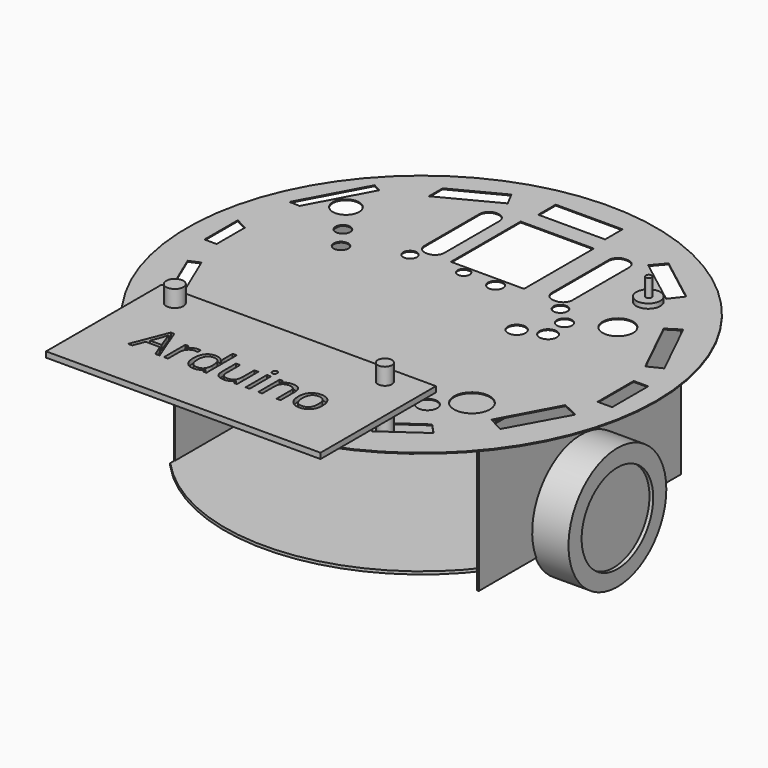
from build123d import *

# Parameters (mm, degrees)
F0_R           = 63.9111702995
F1_DEPTH       = 0.254
F2_W           = 18.2276954874
F2_H           = 5.9562139213
F2_W_2         = 3.9726644754
F2_H_2         = 12.3111242428
F2_W_3         = 18.6114357784
F2_H_3         = 3.4572258592
F2_W_4         = 19.9545305222
F2_H_4         = 23.7919427454
F2_R           = 1.6505332981
F2_R_2         = 2.0396113473
F2_W_5         = 5.3723761812
F2_H_5         = 23.7919408828
F2_W_6         = 5.5642463267
F2_H_6         = 24.3675541133
F2_R_3         = 1.8501413146
F2_R_4         = 1.8832977576
F2_R_5         = 2.0535644144
F2_R_6         = 2.3408672102
F2_R_7         = 2.3992175774
F2_R_8         = 2.0043342178
F2_R_9         = 3.5959734762
F2_R_10        = 1.9777561013
F2_R_11        = 4.047513939
F2_R_12        = 1.9567032502
F2_R_13        = 1.9754290284
F2_R_14        = 4.8842283694
F2_R_15        = 2.6724465659
F2_R_16        = 2.5813546875
F2_R_17        = 4.1507926028
F3_DEPTH       = 53.34
F3_DEPTH_BACK  = 76.454
F4_R           = 3.2674386057
F5_DEPTH       = 1.524
F6_R           = 0.777196863
F7_DEPTH       = 6.35
F8_R           = 2.54
F9_R           = 2.3420782562
F9_R_2         = 1.9282730437
F10_DEPTH      = 15.748
F10_DEPTH_BACK = 2.794
F12_START      = 9.652
F11_W          = 74.8294964433
F11_H          = 39.3334552646
F12_DEPTH      = 1.524
F14_START      = 9.906
F13_TEXT_SIZE  = 13.6177572939
F14_DEPTH      = 10.668
F16_START      = 42.926
F15_W          = 68.8815116882
F15_H          = 37.894424051
F16_DEPTH      = 0.508
F18_START      = -39.37
F17_W          = 69.0733827651
F17_H          = 38.0862951279
F18_DEPTH      = 0.254
F20_START      = 43.18
F19_R          = 16.6703050867
F20_DEPTH      = 10.16
F22_START      = -39.4462
F21_R          = 16.5595980484
F22_DEPTH      = 7.5438
F24_START      = 52.324
F23_R          = 12.195203819
F24_DEPTH      = 51.816
F26_START      = -44.958
F25_R          = 11.3790282157
F26_DEPTH      = 13.208
F28_START      = -33.528
F27_R          = 53.684976613
F28_DEPTH      = 0.762
F30_START      = -29.718
F30_DEPTH      = 27.432
F31_W          = 27.6789963245
F31_H          = 85.5889506638
F32_DEPTH      = 57.658
F32_DEPTH_BACK = 47.244


# Not quite as in the source:
# - Text() gives the source's letters only with a copy of the font that has no kerning and outlines rounded to 1/6400 em; it was checked with that copy


with BuildPart() as f1:
    # F0 (on Top) → F1 (new body)
    with BuildSketch(Plane.XY):
        Circle(F0_R)
    extrude(amount=F1_DEPTH)

    # F2 (on Top) → F3 (cut, two sides)
    with BuildSketch(Plane.XY) as f3_sk:
        with Locations((-0.1918715425, 54.2952399701)):
            Rectangle(F2_W, F2_H)
        Polygon((38.8790406287, 41.5468643842), (26.382194832, 51.1334910989), (23.5169891404, 47.7691923058), (36.192856729, 38.0452337299), align=None)
        Polygon((55.930249393, 12.7593884245), (47.8716939688, 29.2602516711), (44.3243973017, 27.0042982848), (52.1765033906, 10.9261649284), align=None)
        with Locations((56.4382374287, -1.9989344291)):
            Rectangle(F2_W_2, F2_H_2)
        Polygon((46.0938289762, -30.9211090207), (54.4519051909, -15.7124722151), (50.0560939326, -13.6060078889), (41.9458702218, -28.691023613), align=None)
        Polygon((25.3998646187, -48.7983639411), (36.192856729, -41.2095412612), (33.4562764833, -38.2781662047), (23.1152811685, -45.5491786335), align=None)
        with Locations((-0.383741688, -53.8179017603)):
            Rectangle(F2_W_3, F2_H_3)
        Polygon((-42.1155765653, -38.2781662047), (-30.0277341157, -49.5985262096), (-27.4126883596, -45.6261113286), (-38.795024669, -34.7324920255), align=None)
        Polygon((-54.3377436697, -11.8860941993), (-48.9752166669, -24.5263342954), (-46.2652777131, -23.0668127871), (-51.5164032923, -10.6891617167), align=None)
        Polygon((-57.6570853591, 9.3794129285), (-57.6570853591, -2.014640253), (-54.3377436697, -2.014640253), (-54.3377436697, 7.5948205777), align=None)
        Polygon((-44.993635267, 40.1968695223), (-54.3377436697, 22.8168283287), (-51.5164032923, 22.7366536856), (-42.7715001208, 39.0021731772), align=None)
        Polygon((-19.5502191782, 54.9985840917), (-32.8018183124, 48.1027527126), (-32.8018183124, 43.4243921615), (-17.6344756037, 51.3171330094), align=None)
        with Locations((-0.2878075466, 34.6326250583)):
            Rectangle(F2_W_4, F2_H_4)
        with Locations((-5.0845686346, 20.6260792911)):
            Circle(F2_R)
        with Locations((3.933345899, 20.2423390001)):
            Circle(F2_R_2)
        with Locations((-16.5967992507, 34.4407549128)):
            Rectangle(F2_W_5, F2_H_5)
        with Locations((18.2276982814, 34.728561528)):
            Rectangle(F2_W_6, F2_H_6)
        with Locations((-19.0911162645, 19.8585987091)):
            Circle(F2_R_3)
        with Locations((21.5149857104, 20.3715078533)):
            Circle(F2_R_4)
        with Locations((26.1894725263, 15.9154105932)):
            Circle(F2_R_5)
        with Locations((26.7599057406, 9.5835877582)):
            Circle(F2_R_6)
        with Locations((20.2569533139, 7.0166331716)):
            Circle(F2_R_7)
        with Locations((-37.5732146204, 20.0800783932)):
            Circle(F2_R_8)
        with Locations((-43.4749871492, 28.491800651)):
            Circle(F2_R_9)
        with Locations((-33.0960080028, 13.8391247019)):
            Circle(F2_R_10)
        with Locations((-24.6553607285, -30.7952146977)):
            Circle(F2_R_11)
        with Locations((-17.9398916662, -38.0862951279)):
            Circle(F2_R_12)
        with Locations((-5.8520506136, -30.2196051925)):
            Circle(F2_R_13)
        with Locations((33.8651463389, -25.2309720963)):
            Circle(F2_R_14)
        with Locations((26.9578043371, -31.7545682192)):
            Circle(F2_R_15)
        with Locations((20.2423371375, -29.2602516711)):
            Circle(F2_R_16)
        with Locations((36.3594591618, 21.3935598731)):
            Circle(F2_R_17)
    extrude(amount=F3_DEPTH, mode=Mode.SUBTRACT)
    extrude(f3_sk.sketch, amount=-F3_DEPTH_BACK, mode=Mode.SUBTRACT)

    # F4 (on Top) → F5 (join)
    with BuildSketch(Plane.XY):
        with Locations((34.0570136905, 34.6326269209)):
            Circle(F4_R)
    extrude(amount=F5_DEPTH)

    # F6 (on Top) → F7 (join)
    with BuildSketch(Plane.XY):
        with Locations((34.1490767896, 34.6543379128)):
            Circle(F6_R)
    extrude(amount=F7_DEPTH)

    # F8
    f8_edges = [f1.edges().sort_by_distance(p)[0] for p in [
        (15.445575, 46.912339, 0.127),
        (21.009821, 46.912339, 0.127),
        (21.009821, 22.544784, 0.127),
        (15.445575, 22.544784, 0.127),
        (-19.282987, 46.336725, 0.127),
        (-13.910611, 46.336725, 0.127),
        (-19.282987, 22.544784, 0.127),
        (-13.910611, 22.544784, 0.127),
    ]]
    fillet(f8_edges, radius=F8_R)

    # F9 (on Top) → F10 (join, two sides)
    with BuildSketch(Plane.XY) as f10_sk:
        with Locations((-31.1789568514, -45.1855063438)):
            Circle(F9_R)
        with Locations((26.3821929693, -45.5692447722)):
            Circle(F9_R_2)
    extrude(amount=F10_DEPTH)
    extrude(f10_sk.sketch, amount=-F10_DEPTH_BACK)

    # F11 (on Top) → F12 (join)
    with BuildSketch(Plane.XY.offset(F12_START)):
        with Locations((-1.2471601367, -60.0554682314)):
            Rectangle(F11_W, F11_H)
    extrude(amount=F12_DEPTH)

    # F13 (on Top) → F14 (cut)
    with BuildSketch(Plane.XY.offset(F14_START)):
        with Locations((-27.1913576871, -66.1306045949)):
            Text('Arduino', F13_TEXT_SIZE, font='Open Sans', text_align=(TextAlign.LEFT, TextAlign.BOTTOM))
    extrude(amount=F14_DEPTH, mode=Mode.SUBTRACT)

    # F15 (on Right) → F16 (join)
    with BuildSketch(Plane.YZ.offset(F16_START)):
        with Locations((-0.4180036485, -18.9472120255)):
            Rectangle(F15_W, F15_H)
    extrude(amount=F16_DEPTH)

    # F19 (on Right) → F20 (join)
    with BuildSketch(Plane.YZ.offset(F20_START)):
        with Locations((0, -31.1789568514)):
            Circle(F19_R)
    extrude(amount=F20_DEPTH)

    # F23 (on Right) → F24 (cut)
    with BuildSketch(Plane.YZ.offset(F24_START)):
        with Locations((0, -31.3708260655)):
            Circle(F23_R)
    extrude(amount=F24_DEPTH, mode=Mode.SUBTRACT)


with BuildPart() as f18:
    # F17 (on Right) → F18 (new body)
    with BuildSketch(Plane.YZ.offset(F18_START)):
        with Locations((-0.3220681101, -19.0431475639)):
            Rectangle(F17_W, F17_H)
    extrude(amount=-F18_DEPTH)

    # F21 (on Right) → F22 (join)
    with BuildSketch(Plane.YZ.offset(F22_START)):
        with Locations((0, -31.3708260655)):
            Circle(F21_R)
    extrude(amount=-F22_DEPTH)

    # F25 (on Right) → F26 (cut)
    with BuildSketch(Plane.YZ.offset(F26_START)):
        with Locations((0, -31.1789568514)):
            Circle(F25_R)
    extrude(amount=-F26_DEPTH, mode=Mode.SUBTRACT)


with BuildPart() as f28:
    # F27 (on Top) → F28 (new body)
    with BuildSketch(Plane.XY.offset(F28_START)):
        Circle(F27_R)
    extrude(amount=-F28_DEPTH)

    # F29 (on Top) → F30 (cut)
    with BuildSketch(Plane.XY.offset(F30_START)):
        Polygon((43.2554210754, 34.7882919014), (43.18101295, -34.4196464866), (55.0368390977, -34.4196464866), (55.0368390977, 34.7882919014), align=None)
    extrude(amount=-F30_DEPTH, mode=Mode.SUBTRACT)

    # F31 (on Top) → F32 (cut, two sides)
    with BuildSketch(Plane.XY) as f32_sk:
        with Locations((-53.3286035061, -1.4567021281)):
            Rectangle(F31_W, F31_H)
    extrude(amount=-F32_DEPTH, mode=Mode.SUBTRACT)
    extrude(f32_sk.sketch, amount=F32_DEPTH_BACK, mode=Mode.SUBTRACT)


solid = Compound([f1.part, f18.part, f28.part])
